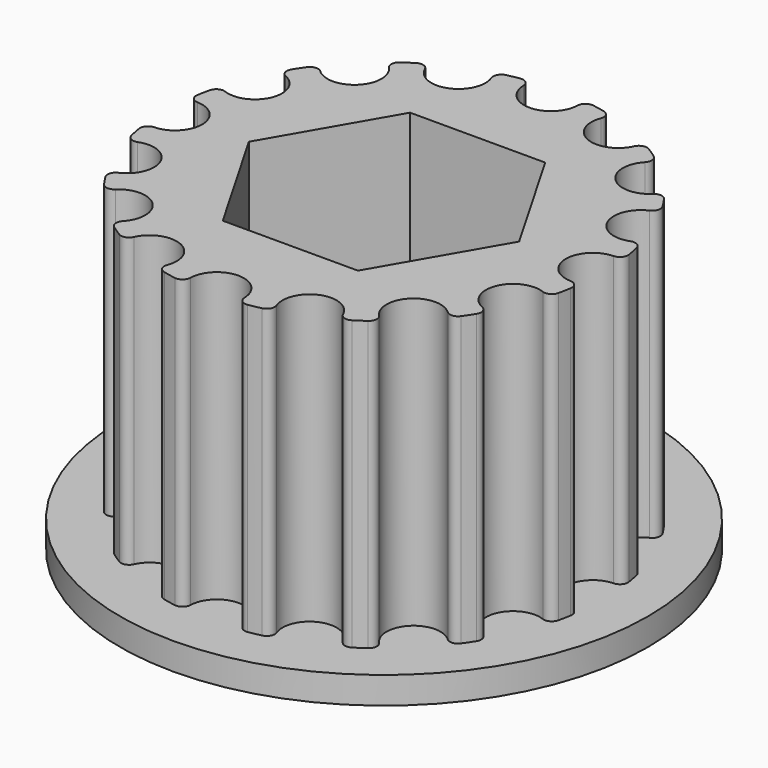
from build123d import *

# Parameters (mm, degrees)
F2_R            = 12.1598954619
F3_DEPTH        = 16
F5_DEPTH        = 16
F5_COPIES_COUNT = 16
F8_R            = 14.6598954619
F8_R_2          = 12.1598954619
F9_DEPTH        = 1.5
F10_DEPTH       = 17.501


# Not quite as in the source:
# - a feature of the source that left no trace in its solid (it failed there, or was rolled back) is left out
# - a pattern or mirror of a feature is missing from the dataset's text; its kind, count and spacing are read off the source's solid


with BuildPart() as f3:
    # F2 (on Top) → F3 (new body)
    with BuildSketch(Plane.XY):
        Circle(F2_R)
    extrude(amount=F3_DEPTH)

    # F4 (on face) → F5 (cut, through all)
    with BuildSketch(Plane.XY.offset(16)):
        with BuildLine():
            ThreePointArc((-2.024177758, 11.9902361131), (-1.6634915573, 11.8941223999), (-1.4994378615, 11.5588333213))
            ThreePointArc((-1.4994378615, 11.5588333213), (0, 10.0998954619), (1.4994378615, 11.5588333213))
            ThreePointArc((1.4994378615, 11.5588333213), (1.6634915573, 11.8941223999), (2.024177758, 11.9902361131))
            ThreePointArc((2.024177758, 11.9902361131), (0, 12.1598954619), (-2.024177758, 11.9902361131))
        make_face()
    f5 = extrude(amount=-F5_DEPTH, mode=Mode.SUBTRACT)

    # F5_copies: F5 ×16 about axis
    f5_copies_axis = Axis((0, 0, 0), (0, 0, 1))
    for i in range(1, F5_COPIES_COUNT):
        add(f5.rotate(f5_copies_axis, i * 360 / F5_COPIES_COUNT), mode=Mode.SUBTRACT)

    # F8 (on face) + F2 (on Top) → F9 (join)
    with BuildSketch(Plane.XY):
        Circle(F8_R)
        Circle(F8_R_2, mode=Mode.SUBTRACT)
    with BuildSketch(Plane.XY):
        Circle(F2_R)
    extrude(amount=-F9_DEPTH)

    # F7 (on face) → F10 (cut, through all)
    with BuildSketch(Plane.XY.offset(16)):
        Polygon((3.7527767497, 6.5), (-3.7527767497, 6.5), (-7.5055534995, 0), (-3.7527767497, -6.5), (3.7527767497, -6.5), (7.5055534995, 0), align=None)
    extrude(amount=-F10_DEPTH, mode=Mode.SUBTRACT)


solid = f3.part
